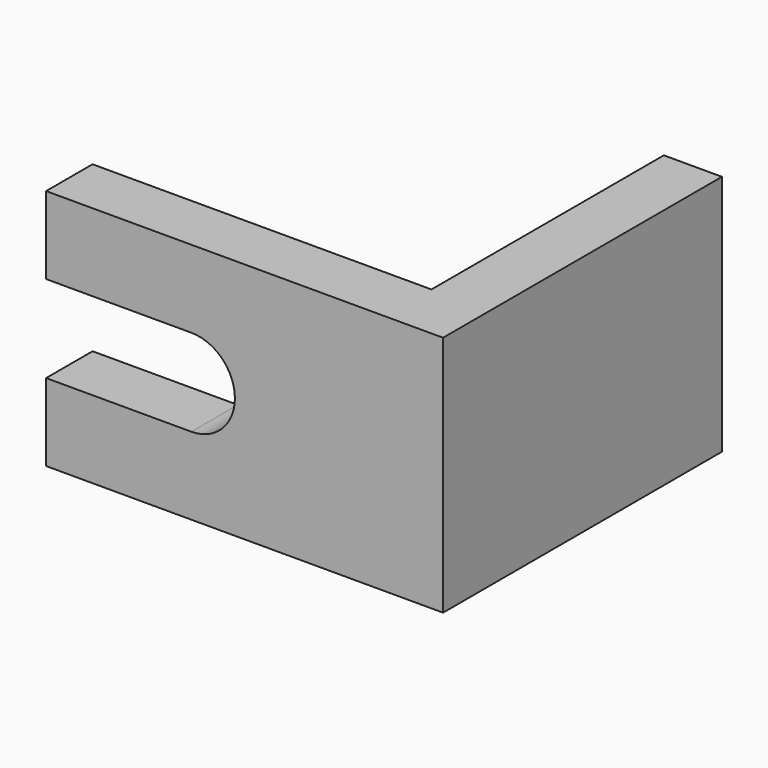
from build123d import *

# Parameters (mm, degrees)
F0_W     = 35
F0_H     = 6
F1_DEPTH = 25
F3_DEPTH = 25
F4_DEPTH = 25


# Not quite as in the source:
# - a feature names something its author has since deleted; it is built from what else it names


with BuildPart() as f1:
    # F0 (on Top) → F1 (new body)
    with BuildSketch(Plane.XY):
        with Locations((-28.5, -30)):
            Rectangle(F0_W, F0_H)
        Polygon((-5, 3), (-11, 3), (-11, -3), (-11, -27), (-11, -33), (-5, -33), (-5, -3), align=None)
    extrude(amount=F1_DEPTH)

    # F2 (on face) → F3 (cut)
    with BuildSketch(Plane(origin=(0, -27, 0), x_dir=(-1, 0, 0), z_dir=(0, 1, 0))):
        with BuildLine():
            ThreePointArc((31, 8), (34.1819805153, 9.3180194847), (35.5, 12.5))
            ThreePointArc((35.5, 12.5), (34.1819805153, 15.6819805153), (31, 17))
            ThreePointArc((31, 17), (26.5, 12.5), (31, 8))
        make_face()
    extrude(amount=-F3_DEPTH, mode=Mode.SUBTRACT)

    # F2 (on face) → F4 (cut)
    with BuildSketch(Plane(origin=(0, -27, 0), x_dir=(-1, 0, 0), z_dir=(0, 1, 0))):
        with BuildLine():
            ThreePointArc((31, 17), (34.1819805153, 15.6819805153), (35.5, 12.5))
            ThreePointArc((35.5, 12.5), (34.1819805153, 9.3180194847), (31, 8))
            Line((31, 8), (46, 8))
            Line((46, 8), (46, 17))
            Line((46, 17), (31, 17))
        make_face()
    extrude(amount=-F4_DEPTH, mode=Mode.SUBTRACT)


solid = f1.part
